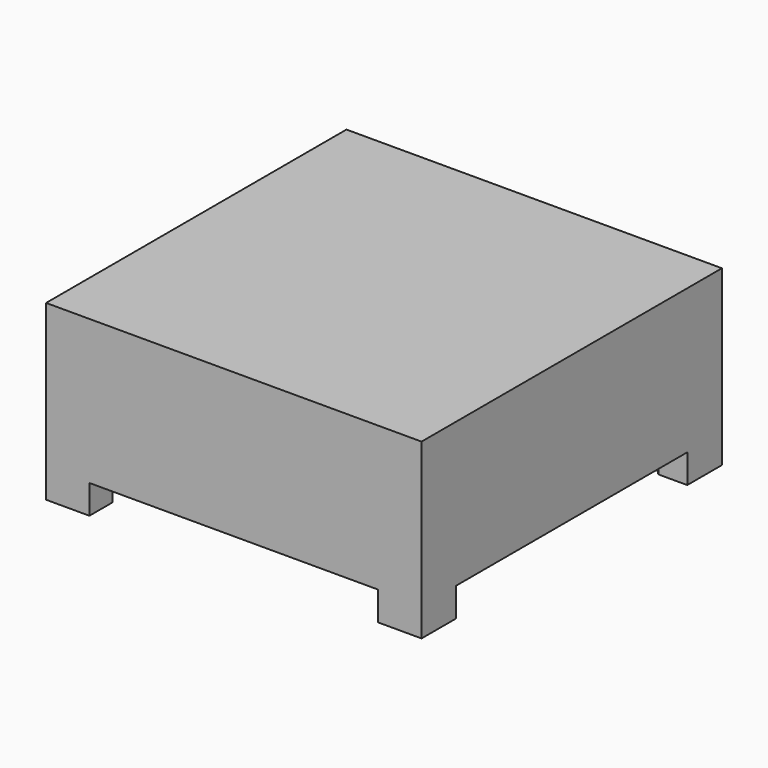
from build123d import *

# Parameters (mm, degrees)
F0_W        = 13
F0_H        = 13
F1_DEPTH    = 6
F2_W        = 10
F2_H        = 10
F3_DEPTH    = 4.5
F4_W        = 10
F4_H        = 2
F5_DEPTH    = 12.5
F6_W        = 10
F6_H        = 2
F7_DEPTH    = 12.5
F8_T1_DEPTH = 2.285841494


# Not quite as in the source:
# - a fillet or chamfer that OpenCascade refuses, or shapes differently, is made with other operations: its cross-section is extruded or revolved along the edge and cut away or added


with BuildPart() as f1:
    # F0 (on Top) → F1 (new body)
    with BuildSketch(Plane.XY):
        Rectangle(F0_W, F0_H)
    extrude(amount=F1_DEPTH)

    # F2 (on Top) → F3 (cut)
    with BuildSketch(Plane.XY):
        Rectangle(F2_W, F2_H)
    extrude(amount=F3_DEPTH, mode=Mode.SUBTRACT)

    # F4 (on Right) → F5 (cut, symmetric)
    with BuildSketch(Plane.YZ):
        Rectangle(F4_W, F4_H)
    extrude(amount=F5_DEPTH, both=True, mode=Mode.SUBTRACT)

    # F6 (on Front) → F7 (cut, symmetric)
    with BuildSketch(Plane.XZ):
        Rectangle(F6_W, F6_H)
    extrude(amount=F7_DEPTH, both=True, mode=Mode.SUBTRACT)

    # F8: chamfer of 0.5 on 4 edges, made by hand

    # F8_s2 → F8_t1 (cut)
    with BuildSketch(Plane.XY.offset(-1.285841494)):
        Polygon((5.5, -5), (5, -5.5), (5, -5), align=None)
        Polygon((5, 5.5), (5.5, 5), (5, 5), align=None)
        Polygon((-5.5, -5), (-5, -5.5), (-5, -5), align=None)
        Polygon((-5, 5.5), (-5.5, 5), (-5, 5), align=None)
    extrude(amount=F8_T1_DEPTH, mode=Mode.SUBTRACT)


solid = f1.part
